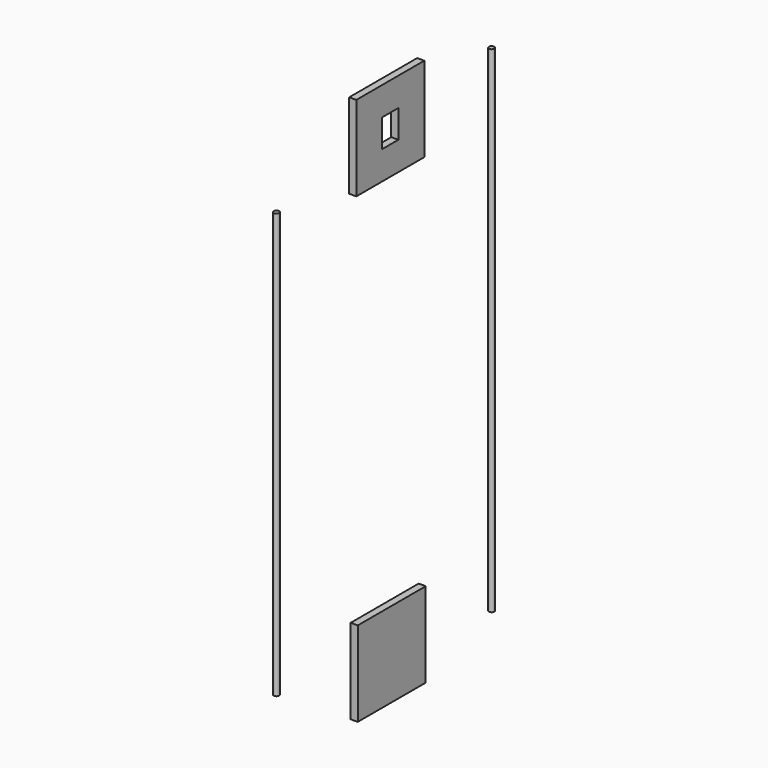
from build123d import *

# Parameters (mm, degrees)
F2_R      = 9.5
F3_DEPTH  = 1500
F9_R      = 9.5
F10_DEPTH = 1750
F13_W     = 300
F13_H     = 300
F13_W_2   = 70.9563016891
F13_H_2   = 98.7522929907
F14_DEPTH = 12.5
F15_W     = 300
F15_H     = 300
F16_DEPTH = 12.5


# Not quite as in the source:
# - the program builds the solid bodies; features that only make, move or delete a surface that nothing else refers to are left out


with BuildPart() as f3:
    # F2 (on Top) → F3 (new body)
    with BuildSketch(Plane.XY):
        Circle(F2_R)
    extrude(amount=-F3_DEPTH)


with BuildPart() as f10:
    # F9 (on offset) → F10 (new body)
    with BuildSketch(Plane.XY.offset(125)):
        with Locations((0, 949.5819807053)):
            Circle(F9_R)
    extrude(amount=-F10_DEPTH)


with BuildPart() as f14:
    # F13 (on Right) → F14 (new body, symmetric)
    with BuildSketch(Plane.YZ):
        with Locations((486.8869185448, 65.7790899277)):
            Rectangle(F13_W, F13_H)
        with Locations((486.8869185448, 65.7790899277)):
            Rectangle(F13_W_2, F13_H_2, mode=Mode.SUBTRACT)
    extrude(amount=F14_DEPTH, both=True)


with BuildPart() as f16:
    # F15 (on Right) → F16 (new body, symmetric)
    with BuildSketch(Plane.YZ):
        with Locations((493.3289289474, -1570.1934099197)):
            Rectangle(F15_W, F15_H)
    extrude(amount=F16_DEPTH, both=True)


solid = Compound([f3.part, f10.part, f14.part, f16.part])
